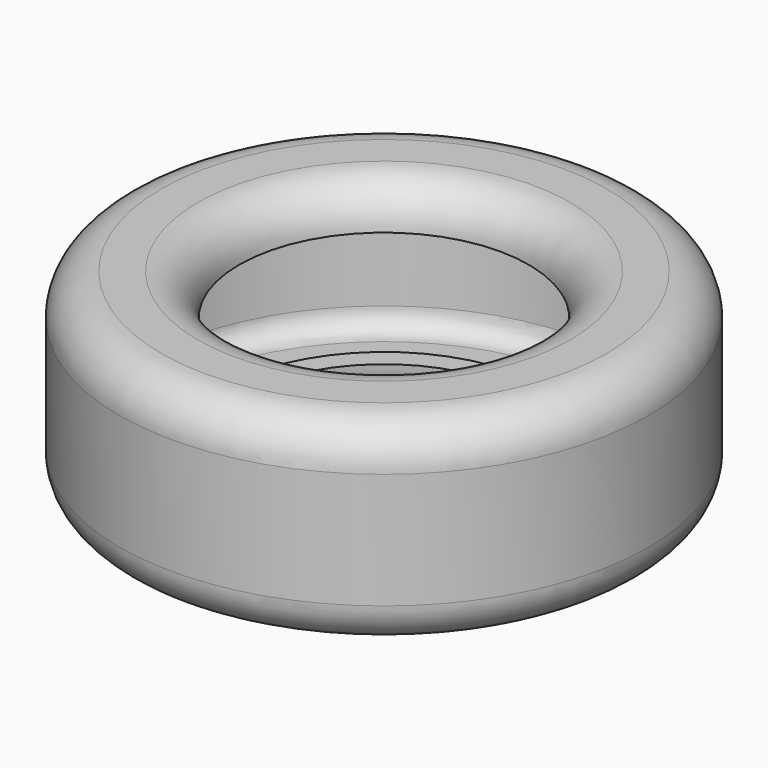
from build123d import *

# Parameters (mm, degrees)
F0_R     = 31.915
F0_R_2   = 17.5
F1_DEPTH = 24
F2_R     = 5
F3_T     = 2.5


# Not quite as in the source:
# - a shell that OpenCascade refuses in one call is made with other operations: the cavity is built on its own and cut out


with BuildPart() as f1:
    # F0 (on Top) → F1 (new body)
    with BuildSketch(Plane.XY):
        Circle(F0_R)
        Circle(F0_R_2, mode=Mode.SUBTRACT)
    extrude(amount=F1_DEPTH)

    # F2
    f2_edges = [f1.edges().sort_by_distance(p)[0] for p in [
        (-31.915, 0, 24),
        (-17.5, 0, 24),
        (-31.915, 0, 0),
        (-17.5, 0, 0),
    ]]
    fillet(f2_edges, radius=F2_R)

    # F3: shell of thickness 2.5, made by hand


with BuildPart() as f3_core1:
    # F3_t2: copy of F1
    add(f1.part)

    # the walls: a layer under each face that stays
    f3_faces = [f3_core1.faces().sort_by_distance(p)[0] for p in [
        (-31.915, 0, 12),
        (-30.4505339059, 0, 1.4644660941),
        (-30.4505339059, 0, 22.5355339059),
        (-17.9433333333, -17.9433333333, 0),
        (-17.9433333333, -17.9433333333, 24),
        (-18.9644660941, 0, 1.4644660941),
        (-18.9644660941, 0, 22.5355339059),
    ]]
    thicken(f3_faces, amount=-F3_T, mode=Mode.SUBTRACT)


with BuildPart() as f1_1:
    add(f1.part)

    # what is left inside the walls is the cavity
    f3_cavity = [f3_core1.part.solids().sort_by_distance(p)[0] for p in [
        (-29.39, 0, 14.333333),
    ]]
    add(f3_cavity, mode=Mode.SUBTRACT)


solid = f1_1.part
